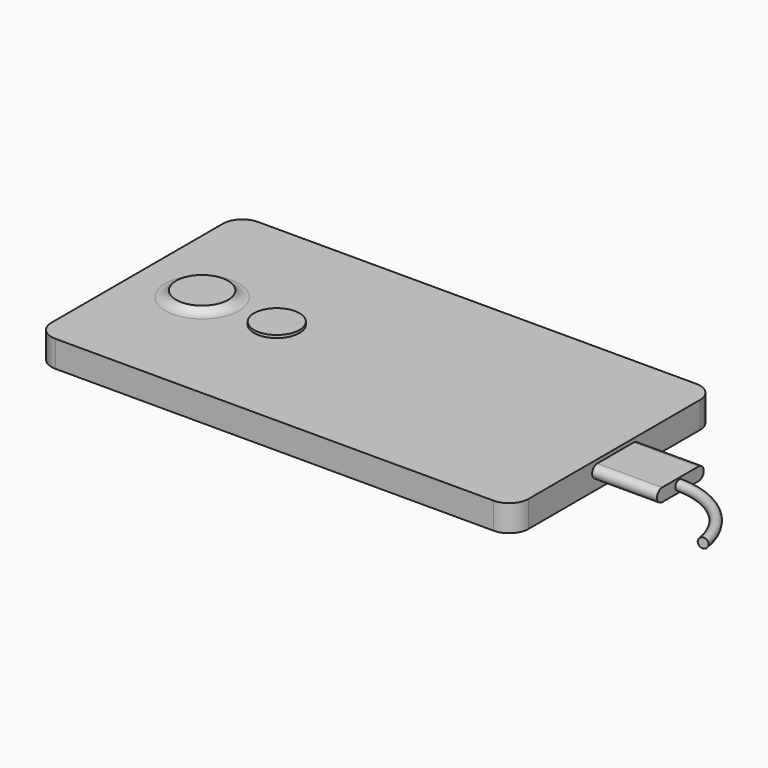
from build123d import *

# Parameters (mm, degrees)
F0_R     = 8
F0_R_2   = 7
F1_DEPTH = 8.15
F2_DEPTH = 10
F3_DEPTH = 9
F5_W     = 115
F5_H     = 65
F6_DEPTH = 0.5
F8_DEPTH = 20
F11_R    = 1.5


# Not quite as in the source:
# - a fillet or chamfer that OpenCascade refuses, or shapes differently, is made with other operations: its cross-section is extruded or revolved along the edge and cut away or added


with BuildPart() as f1:
    # F0 (on Top) → F1 (new body)
    with BuildSketch(Plane.XY):
        with BuildLine():
            Line((-67.5, -39), (67.5, -39))
            ThreePointArc((67.5, -39), (71.7426406871, -37.2426406871), (73.5, -33))
            Line((73.5, -33), (73.5, 33))
            ThreePointArc((73.5, 33), (71.7426406871, 37.2426406871), (67.5, 39))
            Line((67.5, 39), (-67.5, 39))
            ThreePointArc((-67.5, 39), (-71.7426406871, 37.2426406871), (-73.5, 33))
            Line((-73.5, 33), (-73.5, -33))
            ThreePointArc((-73.5, -33), (-71.7426406871, -37.2426406871), (-67.5, -39))
        make_face()
        with Locations((-53.5, 0)):
            Circle(F0_R, mode=Mode.SUBTRACT)
        with Locations((-30.5, 0)):
            Circle(F0_R_2, mode=Mode.SUBTRACT)
        with Locations((-53.5, 0)):
            Circle(F0_R)
        with Locations((-30.5, 0)):
            Circle(F0_R_2)
    extrude(amount=F1_DEPTH)

    # F0 (on Top) → F2 (join)
    with BuildSketch(Plane.XY):
        with Locations((-53.5, 0)):
            Circle(F0_R)
    extrude(amount=F2_DEPTH)

    # F0 (on Top) → F3 (join)
    with BuildSketch(Plane.XY):
        with Locations((-30.5, 0)):
            Circle(F0_R_2)
    extrude(amount=F3_DEPTH)

    # F4: fillet of radius 4 on 1 edges, made by hand

    # F4_s1 → F4_t2 (revolve)
    with BuildSketch(Plane.XZ):
        with BuildLine():
            ThreePointArc((-42.1269450049, 8.15), (-44.0504834111, 8.6428644167), (-45.5, 10))
            Line((-45.5, 10), (-45.5, 8.15))
            Line((-45.5, 8.15), (-42.1269450049, 8.15))
        make_face()
    revolve(axis=Axis((-53.5, 0, 8.15), (0, 0, -1)))

    # F5 (on Top) → F6 (cut)
    with BuildSketch(Plane.XY):
        Rectangle(F5_W, F5_H)
    extrude(amount=F6_DEPTH, mode=Mode.SUBTRACT)

    # F7 (on face) → F8 (join)
    with BuildSketch(Plane.YZ.offset(73.5)):
        with BuildLine():
            ThreePointArc((7.4520160146, 3), (9.4520160146, 5), (7.4520160146, 7))
            Line((7.4520160146, 7), (-6.5479839854, 7))
            ThreePointArc((-6.5479839854, 7), (-8.5479839854, 5), (-6.5479839854, 3))
            Line((-6.5479839854, 3), (7.4520160146, 3))
        make_face()
        with BuildLine():
            ThreePointArc((-1.5, 5), (0, 6.5), (1.5, 5))
            ThreePointArc((1.5, 5), (0, 3.5), (-1.5, 5))
        make_face(mode=Mode.SUBTRACT)
        with BuildLine():
            Line((-1.5, 5), (1.5, 5))
            ThreePointArc((1.5, 5), (0, 6.5), (-1.5, 5))
        make_face()
        with BuildLine():
            ThreePointArc((-1.5, 5), (0, 3.5), (1.5, 5))
            Line((1.5, 5), (-1.5, 5))
        make_face()
    extrude(amount=F8_DEPTH)

    # F12: sweep along a path in F10
    with BuildLine(Plane(origin=(0, 0, 5), x_dir=(1, 0, 0), z_dir=(0, 0, -1))) as f12_path:
        ThreePointArc((93.5, 0), (108.8125986956, 5.7360841116), (116.8597106736, 19.970631121))
    # F11 (on face) → F12 (sweep)
    with BuildSketch(Plane.YZ.offset(93.5)):
        with Locations((0, 5)):
            Circle(F11_R)
    sweep(path=f12_path.line)


solid = f1.part
